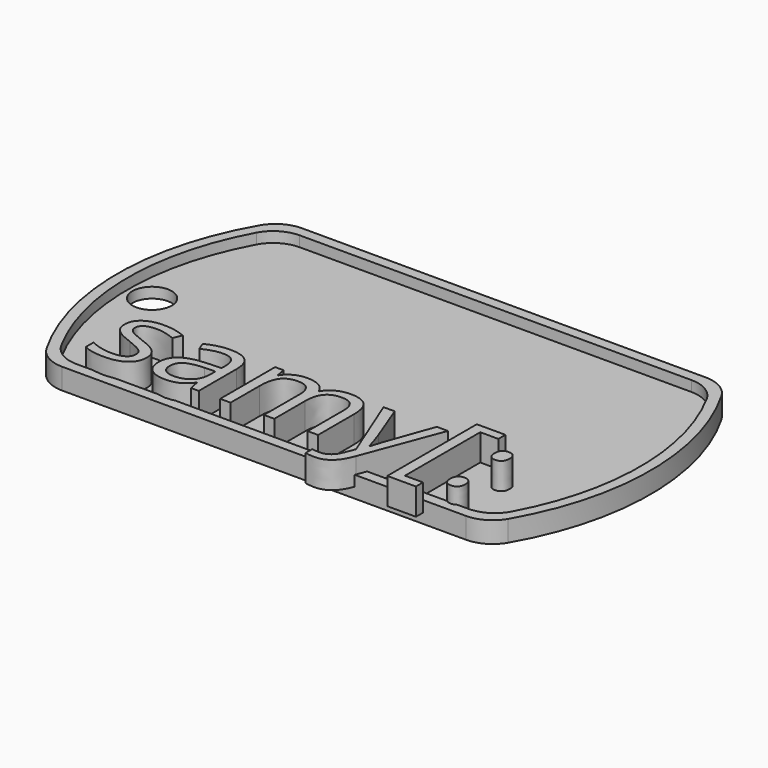
from build123d import *

# Parameters (mm, degrees)
F0_R         = 1.8739594118
F1_DEPTH     = 1
F3_DEPTH     = 1
F4_TEXT_SIZE = 12.2249107516
F5_DEPTH     = 2.54


# Not quite as in the source:
# - Text() gives the source's letters only with a copy of the font that has no kerning and outlines rounded to 1/6400 em; it was checked with that copy


with BuildPart() as f1:
    # F0 (on Top) → F1 (new body)
    with BuildSketch(Plane.XY):
        with BuildLine():
            ThreePointArc((-19.2474145991, 14.2875), (-20.8349145991, 13.862130657), (-21.9970452561, 12.7))
            ThreePointArc((-21.9970452561, 12.7), (-25.4, 0), (-21.9970452561, -12.7))
            ThreePointArc((-21.9970452561, -12.7), (-20.8349145991, -13.862130657), (-19.2474145991, -14.2875))
            Line((-19.2474145991, -14.2875), (19.2474145991, -14.2875))
            ThreePointArc((19.2474145991, -14.2875), (20.8349145991, -13.862130657), (21.9970452561, -12.7))
            ThreePointArc((21.9970452561, -12.7), (25.4, 0), (21.9970452561, 12.7))
            ThreePointArc((21.9970452561, 12.7), (20.8349145991, 13.862130657), (19.2474145991, 14.2875))
            Line((19.2474145991, 14.2875), (-19.2474145991, 14.2875))
        make_face()
        with Locations((-22.0978986472, 0)):
            Circle(F0_R, mode=Mode.SUBTRACT)
    extrude(amount=F1_DEPTH)

    # F2 (on face) → F3 (join)
    with BuildSketch(Plane.XY.offset(1)):
        with BuildLine():
            Line((19.2474145991, 14.2875), (-19.2474145991, 14.2875))
            ThreePointArc((-19.2474145991, 14.2875), (-20.8349145991, 13.862130657), (-21.9970452561, 12.7))
            ThreePointArc((-21.9970452561, 12.7), (-25.4, 0), (-21.9970452561, -12.7))
            ThreePointArc((-21.9970452561, -12.7), (-20.8349145991, -13.862130657), (-19.2474145991, -14.2875))
            Line((-19.2474145991, -14.2875), (19.2474145991, -14.2875))
            ThreePointArc((19.2474145991, -14.2875), (20.8349145991, -13.862130657), (21.9970452561, -12.7))
            ThreePointArc((21.9970452561, -12.7), (25.4, 0), (21.9970452561, 12.7))
            ThreePointArc((21.9970452561, 12.7), (20.8349145991, 13.862130657), (19.2474145991, 14.2875))
        make_face()
        with BuildLine():
            ThreePointArc((-21.4526124879, 11.6252061249), (-20.2856017842, 12.8404540819), (-18.6611352482, 13.2875))
            Line((-18.6611352482, 13.2875), (18.6611352482, 13.2875))
            ThreePointArc((18.6611352482, 13.2875), (20.2856017842, 12.8404540819), (21.4526124879, 11.6252061249))
            ThreePointArc((21.4526124879, 11.6252061249), (24.4, 0), (21.4526124879, -11.6252061249))
            ThreePointArc((21.4526124879, -11.6252061249), (20.2856017842, -12.8404540819), (18.6611352482, -13.2875))
            Line((18.6611352482, -13.2875), (-18.6611352482, -13.2875))
            ThreePointArc((-18.6611352482, -13.2875), (-20.2856017842, -12.8404540819), (-21.4526124879, -11.6252061249))
            ThreePointArc((-21.4526124879, -11.6252061249), (-24.4, 0), (-21.4526124879, 11.6252061249))
        make_face(mode=Mode.SUBTRACT)
    extrude(amount=F3_DEPTH)


with BuildPart() as f5:
    # F4 (on face) → F5 (new body)
    with BuildSketch(Plane.XY.offset(1)):
        with Locations((-18.6611352482, -13.2875)):
            Text('samy[:', F4_TEXT_SIZE, font='Open Sans', text_align=(TextAlign.LEFT, TextAlign.BOTTOM))
    extrude(amount=F5_DEPTH)


solid = Compound([f1.part, f5.part])
